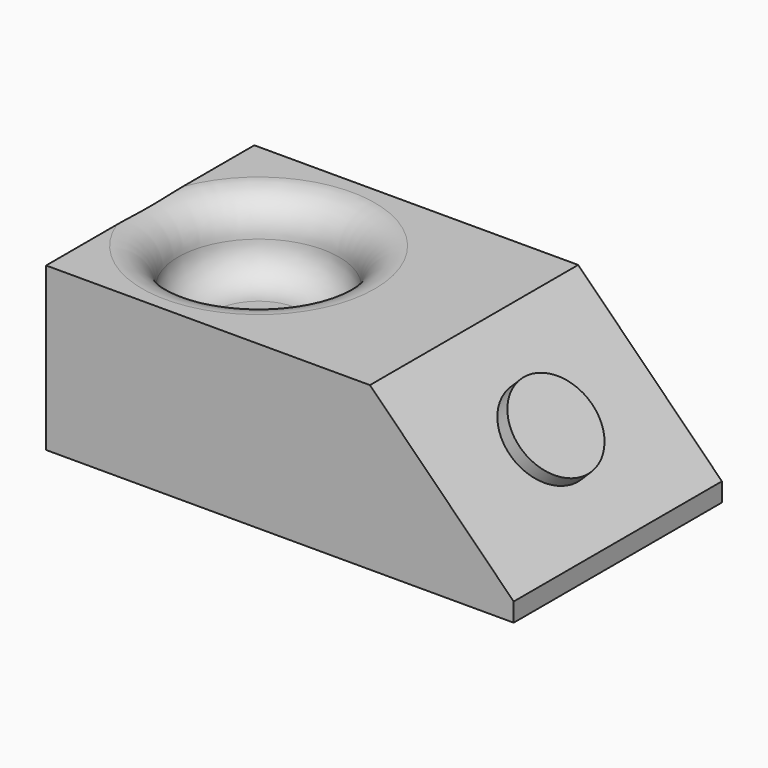
from build123d import *

# Parameters (mm, degrees)
F0_W     = 165.2496345341
F0_H     = 91.986246407
F1_DEPTH = 57.404
F2_R     = 28.4210411612
F3_DEPTH = 25.4
F5_SIZE  = 50.8
F6_R     = 16.0842611484
F7_DEPTH = 5


# Not quite as in the source:
# - a fillet or chamfer that OpenCascade refuses, or shapes differently, is made with other operations: its cross-section is extruded or revolved along the edge and cut away or added


with BuildPart() as f1:
    # F0 (on Top) → F1 (new body)
    with BuildSketch(Plane.XY):
        with Locations((-43.7887068838, 9.0369544923)):
            Rectangle(F0_W, F0_H)
    extrude(amount=F1_DEPTH)

    # F2 (on face) → F3 (cut)
    with BuildSketch(Plane.XY.offset(57.404)):
        with Locations((-87.9544317722, 8.8456757367)):
            Circle(F2_R)
    extrude(amount=-F3_DEPTH, mode=Mode.SUBTRACT)

    # F4: fillet of radius 12.7 on 2 edges, made by hand

    # F4_s1 → F4_t2 (revolve)
    with BuildSketch(Plane.XZ.offset(-8.8456757367)):
        with BuildLine():
            ThreePointArc((-59.5333906111, 44.704), (-63.25313449, 35.7237438789), (-72.2333906111, 32.004))
            Line((-72.2333906111, 32.004), (-59.5333906111, 32.004))
            Line((-59.5333906111, 32.004), (-59.5333906111, 44.704))
        make_face()
    revolve(axis=Axis((-87.9544317722, 8.8456757367, 32.004), (0, 0, 1)))

    # F4_s3 → F4_t4 (revolve, cut)
    with BuildSketch(Plane.XZ.offset(-8.8456757367)):
        with BuildLine():
            ThreePointArc((-46.8333906111, 57.404), (-55.8136467322, 53.6842561211), (-59.5333906111, 44.704))
            Line((-59.5333906111, 44.704), (-59.5333906111, 57.404))
            Line((-59.5333906111, 57.404), (-46.8333906111, 57.404))
        make_face()
    revolve(axis=Axis((-87.9544317722, 8.8456757367, 57.404), (0, 0, 1)), mode=Mode.SUBTRACT)

    # F5
    f5_edges = [f1.edges().sort_by_distance(p)[0] for p in [
        (38.83611, 9.036954, 57.404),
    ]]
    chamfer(f5_edges, length=F5_SIZE)

    # F6 (on face) → F7 (join)
    with BuildSketch(Plane(origin=(22.7200551916, 0, 22.7200551916), x_dir=(0, 1, 0), z_dir=(0.7071067812, 0, 0.7071067812))):
        with Locations((9.0369544923, 13.1294806603)):
            Circle(F6_R)
    extrude(amount=F7_DEPTH)


solid = f1.part
